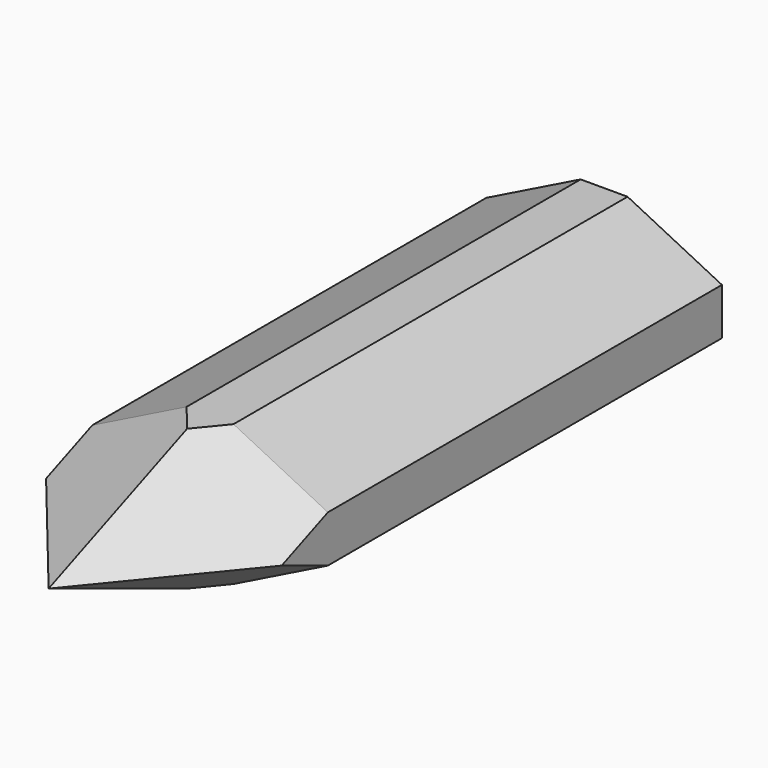
from build123d import *

# Parameters (mm, degrees)
F1_DEPTH    = 762
F2_T1_DEPTH = 1300.1781500313
F2_T3_DEPTH = 1300.1781500313
F2_T5_DEPTH = 1300.1781500313
F2_T7_DEPTH = 1300.1781500313


# Not quite as in the source:
# - a fillet or chamfer that OpenCascade refuses, or shapes differently, is made with other operations: its cross-section is extruded or revolved along the edge and cut away or added


with BuildPart() as f1:
    # F0 (on Front) → F1 (new body)
    with BuildSketch(Plane.XZ):
        Polygon((25.4, 76.2), (0, 76.2), (-25.4, 76.2), (-127.5811195374, 25.4), (-127.5811195374, 0), (-127.5811195374, -25.4), (-25.4, -76.2), (0, -76.2), (25.4, -76.2), (127.5811195374, -25.4), (127.5811195374, 0), (127.5811195374, 25.4), align=None)
    extrude(amount=F1_DEPTH)

    # F2: chamfer of 228.6 x 83.2035955533 on 4 edges, made by hand

    # F2_s2 → F2_t1 (cut)
    with BuildSketch(Plane(origin=(541.036756959, 0, 268.9798993978), x_dir=(0, 1, 0), z_dir=(-0.8954433759, 0, -0.4451754267))):
        Polygon((-762, 3.6633544712), (-533.4, -79.540241082), (-762, -79.540241082), align=None)
    extrude(amount=F2_T1_DEPTH, mode=Mode.SUBTRACT)

    # F2_s4 → F2_t3 (cut)
    with BuildSketch(Plane(origin=(623.1991549624, 0, -309.8274633849), x_dir=(0, 1, 0), z_dir=(-0.8954433759, 0, 0.4451754267))):
        Polygon((-533.4, -79.540241082), (-762, 3.6633544712), (-762, -79.540241082), align=None)
    extrude(amount=F2_T3_DEPTH, mode=Mode.SUBTRACT)

    # F2_s6 → F2_t5 (cut)
    with BuildSketch(Plane(origin=(-541.036756959, 0, -268.9798993978), x_dir=(0, 1, 0), z_dir=(0.8954433759, 0, 0.4451754267))):
        Polygon((-762, 3.6633544712), (-533.4, -79.540241082), (-762, -79.540241082), align=None)
    extrude(amount=F2_T5_DEPTH, mode=Mode.SUBTRACT)

    # F2_s8 → F2_t7 (cut)
    with BuildSketch(Plane(origin=(-623.1991549624, 0, 309.8274633849), x_dir=(0, 1, 0), z_dir=(0.8954433759, 0, -0.4451754267))):
        Polygon((-762, 3.6633544712), (-533.4, -79.540241082), (-762, -79.540241082), align=None)
    extrude(amount=F2_T7_DEPTH, mode=Mode.SUBTRACT)


solid = f1.part
